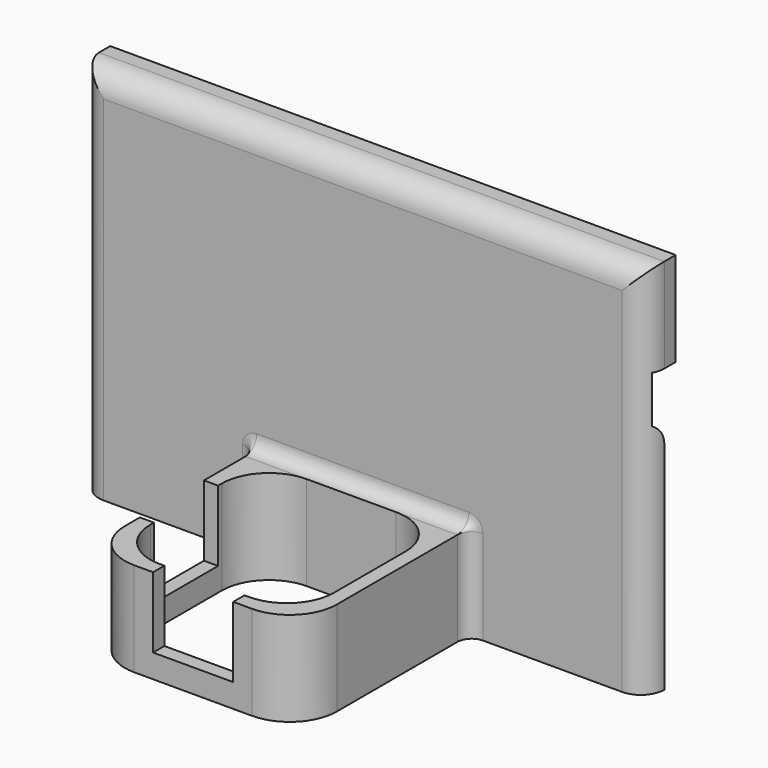
from build123d import *

# Parameters (mm, degrees)
F1_DEPTH     = 20
F2_W         = 17
F2_H         = 15
F3_DEPTH     = 5
F4_W         = 17
F4_H         = 15
F5_DEPTH     = 5
F6_W         = 120
F6_H         = 80
F7_DEPTH     = 5
F9_DEPTH     = 20
F11_DEPTH    = 45
F14_R        = 4.99999
F15_W        = 120
F15_H        = 10
F16_DEPTH    = 2.5
F17_DEPTH    = 3
F18_T1_DEPTH = 141.6506350946


# Not quite as in the source:
# - a fillet or chamfer that OpenCascade refuses, or shapes differently, is made with other operations: its cross-section is extruded or revolved along the edge and cut away or added
# - a fillet or chamfer is up to 0.001 mm smaller than in the source, because OpenCascade refuses the exact size


with BuildPart() as f1:
    # F0 (on Top) → F1 (new body)
    with BuildSketch(Plane.XY):
        with BuildLine():
            Line((8.9493141696, 27.1629239851), (-36.0506858304, 27.1629239851))
            Line((-36.0506858304, 27.1629239851), (-36.0506858304, -7.8370760149))
            ThreePointArc((-36.0506858304, -7.8370760149), (-33.1217536423, -14.9081438267), (-26.0506858304, -17.8370760149))
            Line((-26.0506858304, -17.8370760149), (-1.0506858304, -17.8370760149))
            ThreePointArc((-1.0506858304, -17.8370760149), (6.0203819815, -14.9081438267), (8.9493141696, -7.8370760149))
            Line((8.9493141696, -7.8370760149), (8.9493141696, 27.1629239851))
        make_face()
        with BuildLine():
            ThreePointArc((-33.0506858304, 14.1629239851), (-30.1217536423, 21.233991797), (-23.0506858304, 24.1629239851))
            Line((-23.0506858304, 24.1629239851), (-4.0506858304, 24.1629239851))
            ThreePointArc((-4.0506858304, 24.1629239851), (3.0203819815, 21.233991797), (5.9493141696, 14.1629239851))
            Line((5.9493141696, 14.1629239851), (5.9493141696, -4.8370760149))
            ThreePointArc((5.9493141696, -4.8370760149), (3.0203819815, -11.9081438267), (-4.0506858304, -14.8370760149))
            Line((-4.0506858304, -14.8370760149), (-23.0506858304, -14.8370760149))
            ThreePointArc((-23.0506858304, -14.8370760149), (-30.1217536423, -11.9081438267), (-33.0506858304, -4.8370760149))
            Line((-33.0506858304, -4.8370760149), (-33.0506858304, 14.1629239851))
        make_face(mode=Mode.SUBTRACT)
    extrude(amount=F1_DEPTH)

    # F2 (on face) → F3 (cut)
    with BuildSketch(Plane.XZ.offset(17.8370760149)):
        with Locations((-13.5506858304, 12.5)):
            Rectangle(F2_W, F2_H)
    extrude(amount=-F3_DEPTH, mode=Mode.SUBTRACT)

    # F4 (on face) → F5 (cut)
    with BuildSketch(Plane(origin=(-36.0506858304, 0, 0), x_dir=(0, -1, 0), z_dir=(-1, 0, 0))):
        with Locations((-4.6629239851, 12.5)):
            Rectangle(F4_W, F4_H)
    extrude(amount=-F5_DEPTH, mode=Mode.SUBTRACT)

    # F6 (on face) → F7 (join)
    with BuildSketch(Plane(origin=(0, 27.1629239851, 0), x_dir=(-1, 0, 0), z_dir=(0, 1, 0))):
        with Locations((13.5506858304, 40)):
            Rectangle(F6_W, F6_H)
    extrude(amount=F7_DEPTH)

    # F8 (on face) → F9 (join)
    with BuildSketch(Plane(origin=(0, 0, 0), x_dir=(1, 0, 0), z_dir=(0, 0, -1))):
        with BuildLine():
            ThreePointArc((-36.0506858304, -24.1629239851), (-36.9293654869, -26.2842443287), (-39.0506858304, -27.1629239851))
            Line((-39.0506858304, -27.1629239851), (-36.0506858304, -27.1629239851))
            Line((-36.0506858304, -27.1629239851), (-36.0506858304, -24.1629239851))
        make_face()
        with BuildLine():
            Line((8.9493141696, -27.1629239851), (11.9493141696, -27.1629239851))
            ThreePointArc((11.9493141696, -27.1629239851), (9.827993826, -26.2842443287), (8.9493141696, -24.1629239851))
            Line((8.9493141696, -24.1629239851), (8.9493141696, -27.1629239851))
        make_face()
    extrude(amount=-F9_DEPTH)

    # F10 (on face) → F11 (join)
    with BuildSketch(Plane.YZ.offset(8.9493141696)):
        with BuildLine():
            ThreePointArc((27.1629239851, 23), (26.2842443287, 20.8786796564), (24.1629239851, 20))
            Line((24.1629239851, 20), (27.1629239851, 20))
            Line((27.1629239851, 20), (27.1629239851, 23))
        make_face()
    extrude(amount=-F11_DEPTH)

    # F11_face (on face) → F12 (revolve)
    with BuildSketch(Plane(origin=(8.9493141696, 26.4928201683, 20.6701038168), x_dir=(0, 1, 0), z_dir=(1, 0, 0))):
        with BuildLine():
            ThreePointArc((0.6701038168, 2.3298961832), (-0.2085758396, 0.2085758396), (-2.3298961832, -0.6701038168))
            Line((-2.3298961832, -0.6701038168), (0.6701038168, -0.6701038168))
            Line((0.6701038168, -0.6701038168), (0.6701038168, 2.3298961832))
        make_face()
    revolve(axis=Axis((8.9493141696, 25.6629239851, 20), (0, 1, 0)))

    # F11_face1 (on face) → F13 (revolve)
    with BuildSketch(Plane(origin=(-36.0506858304, 26.4928201683, 20.6701038168), x_dir=(0, 1, 0), z_dir=(-1, 0, 0))):
        with BuildLine():
            ThreePointArc((-2.3298961832, 0.6701038168), (-0.2085758396, -0.2085758396), (0.6701038168, -2.3298961832))
            Line((0.6701038168, -2.3298961832), (0.6701038168, 0.6701038168))
            Line((0.6701038168, 0.6701038168), (-2.3298961832, 0.6701038168))
        make_face()
    revolve(axis=Axis((-36.0506858304, 25.6629239851, 20), (0, 1, 0)))

    # F14 (radius 5 in the source; OpenCascade refuses exactly that, so slightly less here)
    f14_edges = [f1.edges().sort_by_distance(p)[0] for p in [
        (-73.550686, 27.162924, 40),
        (-13.550686, 27.162924, 80),
        (46.449314, 27.162924, 40),
    ]]
    fillet(f14_edges, radius=F14_R)

    # F15 (on face) → F16 (cut)
    with BuildSketch(Plane(origin=(0, 32.1629239851, 0), x_dir=(-1, 0, 0), z_dir=(0, 1, 0))):
        with Locations((13.5506858304, 55)):
            Rectangle(F15_W, F15_H)
    extrude(amount=-F16_DEPTH, mode=Mode.SUBTRACT)

    # F17 (add): a face of the model
    f17_faces = [f1.faces().sort_by_distance(p)[0] for p in [
        (-13.5506858304, 32.1629239851, 70),
    ]]
    extrude(f17_faces, amount=F17_DEPTH)

    # F18: fillet of radius 5 on 5 edges, made by hand

    # F18_s2 → F18_t1 (cut)
    with BuildSketch(Plane.YZ.offset(-84.3760033777)):
        with BuildLine():
            ThreePointArc((29.6629239851, 50), (31.4930510041, 48.1698729811), (32.1629239851, 45.6698729811))
            Line((32.1629239851, 45.6698729811), (32.1629239851, 50))
            Line((32.1629239851, 50), (29.6629239851, 50))
        make_face()
    extrude(amount=F18_T1_DEPTH, mode=Mode.SUBTRACT)


solid = f1.part
